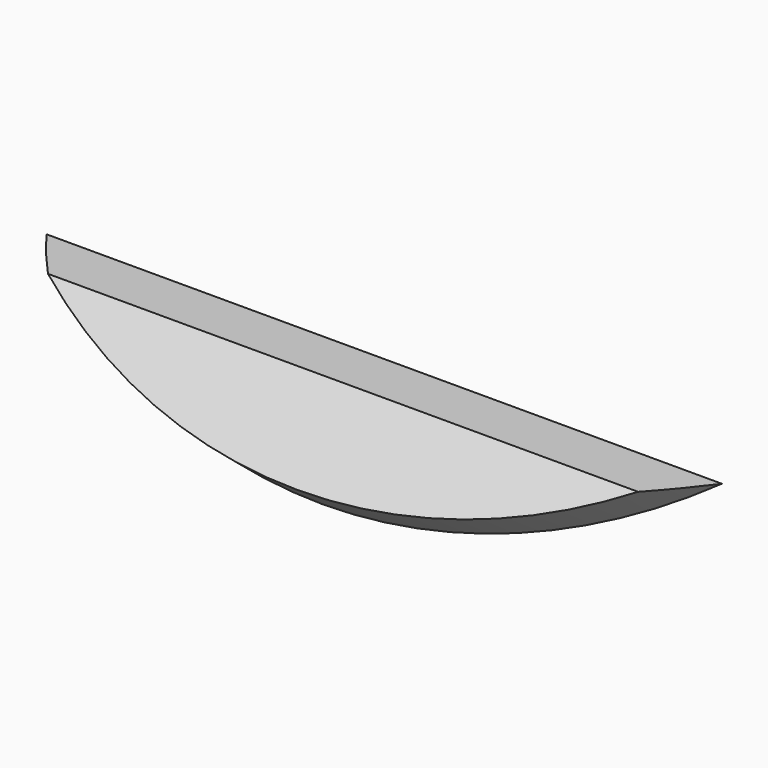
from build123d import *

# Parameters (mm, degrees)
F1_DEPTH = 25.4
F3_DEPTH = 31.75
F5_DEPTH = 25.4
F6_W     = 25.4
F6_H     = 270.2104524793
F7_DEPTH = 508


with BuildPart() as f1:
    # F0 (on Right) → F1 (new body)
    with BuildSketch(Plane.YZ):
        Polygon((27.3959822953, -102.7910036798), (27.3959822953, 85.8886760547), (-43.5209119504, 143.3160446986), (-242.814470184, -102.7910036798), align=None)
    extrude(amount=F1_DEPTH)

    # F6 (on face) → F7 (cut)
    with BuildSketch(Plane(origin=(0, 0, -102.7910036798), x_dir=(1, 0, 0), z_dir=(0, 0, -1))):
        with Locations((12.7, 107.7092439444)):
            Rectangle(F6_W, F6_H)
    extrude(amount=-F7_DEPTH, mode=Mode.SUBTRACT)


with BuildPart() as f3:
    # F2 (on face) → F3 (new body)
    with BuildSketch(Plane(origin=(0, -96.3768318043, 78.044419565), x_dir=(1, 0, 0), z_dir=(0, -0.7771459615, 0.629320391))):
        with BuildLine():
            Line((0, -232.6917107126), (-255.0972491243, -232.6917107126))
            ThreePointArc((-255.0972491243, -232.6917107126), (12.7, -330.742311978), (280.4972491243, -232.6917107126))
            Line((280.4972491243, -232.6917107126), (25.4, -232.6917107126))
            Line((25.4, -232.6917107126), (12.7, -232.6917107126))
            Line((12.7, -232.6917107126), (0, -232.6917107126))
        make_face()
    extrude(amount=F3_DEPTH)

    # F4 (on face) → F5 (cut)
    with BuildSketch(Plane(origin=(0, 0, -102.7910036798), x_dir=(1, 0, 0), z_dir=(0, 0, -1))):
        Polygon((0, 242.814470184), (12.7, 242.814470184), (25.4, 242.814470184), (293.8941717148, 242.814470184), (293.8941717148, 285.4833602905), (-263.440400362, 285.4833602905), (-263.440400362, 242.814470184), align=None)
    extrude(amount=-F5_DEPTH, mode=Mode.SUBTRACT)


solid = f3.part
